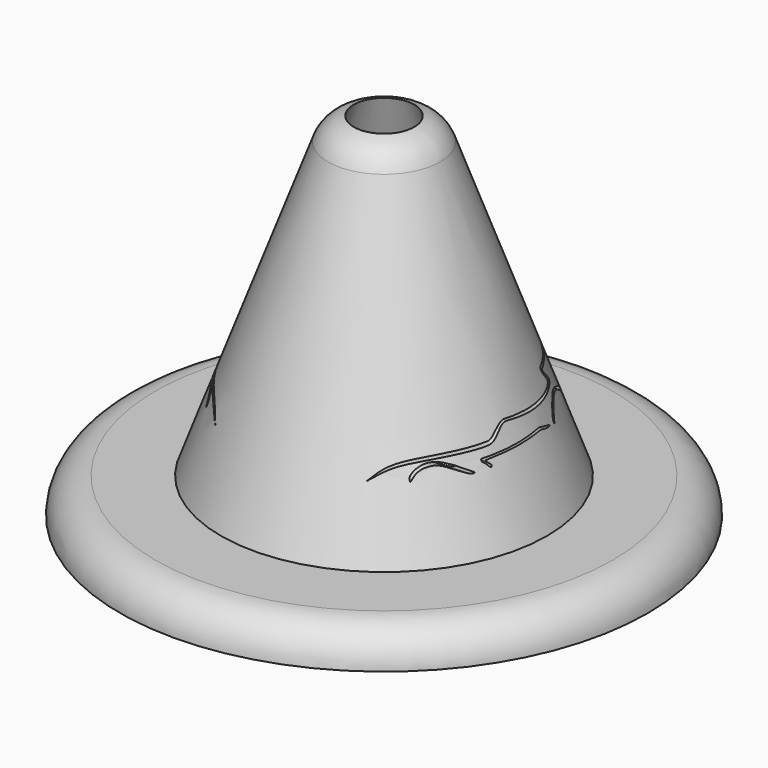
from build123d import *

# Parameters (mm, degrees)
F0_R          = 50
F0_R_2        = 45
F1_DEPTH      = 100
F1_TAPER      = 20
F2_DEPTH      = 100
F2_TAPER      = 20
F0_R_3        = 75
F3_DEPTH      = 10
F3_TAPER      = -20
F5_DEPTH      = 40
F5_DEPTH_BACK = 40


# Not quite as in the source:
# - a fillet or chamfer that OpenCascade refuses, or shapes differently, is made with other operations: its cross-section is extruded or revolved along the edge and cut away or added


with BuildPart() as f1:
    # F0 (on Top) → F1 (new body)
    with BuildSketch(Plane.XY):
        Circle(F0_R)
        Circle(F0_R_2, mode=Mode.SUBTRACT)
        Circle(F0_R_2)
    extrude(amount=F1_DEPTH, taper=F1_TAPER)

    # F0 (on Top) → F2 (cut)
    with BuildSketch(Plane.XY):
        Circle(F0_R_2)
    extrude(amount=F2_DEPTH, taper=F2_TAPER, mode=Mode.SUBTRACT)

    # F0 (on Top) → F3 (join)
    with BuildSketch(Plane.XY):
        Circle(F0_R_3)
        Circle(F0_R, mode=Mode.SUBTRACT)
    extrude(amount=F3_DEPTH, taper=F3_TAPER)

    # F4 (on Right) → F5 (cut, two sides)
    with BuildSketch(Plane.YZ) as f5_sk:
        with BuildLine():
            add(Edge.make_bspline(
                [(-33.0905122474, 29.0107644992), (-32.4736289516, 29.4855445157), (-31.0186418233, 30.6053652357), (-26.9459934351, 33.0948601121), (-14.7801623352, 33.2154481172), (-8.672900368, 33.0818885283), (-7.3010598226, 33.623406531), (-5.7671409301, 34.7695034497), (-3.603350549, 36.7572104234), (-1.1111195238, 36.4115912996), (5.5015940536, 35.4228440969), (10.74246847, 35.0882430818), (15.6437072481, 34.987577792), (20.8910014478, 35.7164902028), (18.1980442225, 37.9974433258), (16.9738401589, 39.7907033697), (17.7865173787, 39.7330347723), (20.0394734839, 39.7776412616), (26.3179551973, 39.6554872999), (30.4444185386, 40.2482755124), (32.5263710484, 40.5470123977)],
                knots=[0, 0, 0, 0, 0.0451475883, 0.1069196297, 0.2094003196, 0.2800605832, 0.3124517037, 0.3521408548, 0.3999822498, 0.4445315809, 0.5189515251, 0.5865582039, 0.6536105299, 0.7088728063, 0.7541204751, 0.7934668639, 0.8112489161, 0.8536560226, 0.926473828, 1, 1, 1, 1], degree=3))
            add(Edge.make_bspline(
                [(32.5263710484, 40.5470123977), (30.1976356747, 40.4635342007), (25.2690463426, 40.2868590164), (19.4529417348, 40.396089847), (16.3849193114, 40.4537096218)],
                knots=[0, 0, 0, 0, 0.472495316, 1, 1, 1, 1], degree=3))
            add(Edge.make_bspline(
                [(16.3849193114, 40.4537096218), (16.5686048113, 39.7383730029), (16.9565205292, 38.3150686964), (21.4343349953, 34.8701721906), (7.4818398942, 35.9873174196), (-3.2351667173, 37.2132535267)],
                knots=[0, 0, 0, 0, 0.1993748097, 0.391377201, 1, 1, 1, 1], degree=3))
            add(Edge.make_bspline(
                [(-3.2351667173, 37.2132535267), (-5.9701177432, 36.3668073114), (-6.9092386051, 34.5355377436), (-8.6203338758, 34.1090930525)],
                knots=[0, 0, 0, 0, 6.2157732885, 6.2157732885, 6.2157732885, 6.2157732885], degree=3))
            add(Edge.make_bspline(
                [(-8.6203338758, 34.1090930525), (-14.5863803397, 33.8637664695), (-27.6658774108, 34.5977789594), (-31.4557963438, 30.6431434265), (-33.0905122474, 29.0107644992)],
                knots=[0, 0, 0, 0, 0.618362291, 1, 1, 1, 1], degree=3))
        make_face()
        with BuildLine():
            add(Edge.make_bspline(
                [(-26.909318541, 28.6785699918), (-26.8956395308, 29.0550856543), (-26.8601785209, 30.0311523057), (-24.3210936276, 32.293186642), (-20.5030238961, 32.9063750111), (-16.421347657, 30.179098201), (-13.9781577953, 28.5466181457)],
                knots=[0, 0, 0, 0, 0.1464289315, 0.3795974805, 0.6286424848, 1, 1, 1, 1], degree=3))
            add(Edge.make_bspline(
                [(-13.9781577953, 28.5466181457), (-14.2737865515, 28.4716503343), (-15.2163200417, 28.2326354499), (-19.7471855154, 31.2612430572), (-22.0542026714, 31.9048500684), (-25.0846623627, 31.1021368623), (-26.2937481092, 29.4961903866), (-26.909318541, 28.6785699918)],
                knots=[0, 0, 0, 0, 0.1254845549, 0.4000740558, 0.5918971887, 0.7922264616, 1, 1, 1, 1], degree=3))
        make_face()
        with BuildLine():
            add(Edge.make_bspline(
                [(-9.9345830013, 28.6598701102), (-10.2675818403, 28.7198319859), (-10.9003286687, 29.9244436138), (-11.7667029195, 30.1550577471), (-11.7303005199, 30.9825030934), (-11.1805494134, 30.9455152519), (7.8860175685, 31.2394349499), (7.5029550194, 31.2710197722), (13.3797988078, 29.5980368417), (11.1528119969, 29.6089395606), (8.1590386099, 30.5150460799), (7.7765984584, 30.6470446813), (-10.7555014846, 30.5645954508), (-10.7132201965, 30.3452443993), (-10.7949253185, 30.0675032085), (-9.2597765347, 29.0612951912), (-9.7549917724, 28.6275317784), (-9.9345830013, 28.6598701102)],
                knots=[0, 0, 0, 0, 0.0574162707, 0.1006189695, 0.1351088035, 0.168735216, 0.3685417337, 0.4055091331, 0.5050900385, 0.5473015241, 0.628784027, 0.6826490599, 0.8788117099, 0.8897597101, 0.9105480692, 0.9690345509, 1, 1, 1, 1], degree=3))
        make_face()
        with BuildLine():
            add(Edge.make_bspline(
                [(14.7013281602, 28.6206390895), (14.6405472638, 29.0722058099), (14.4989867185, 30.1239183553), (16.2352054341, 32.0087749061), (18.8620217309, 33.7182216009), (21.9139736425, 33.7315879037), (26.9762607989, 30.6280239128), (30.3145315813, 28.5814120411)],
                knots=[0, 0, 0, 0, 0.126477424, 0.2945697447, 0.4823409145, 0.6586352874, 1, 1, 1, 1], degree=3))
            add(Edge.make_bspline(
                [(14.7013281602, 28.6206390895), (14.8536817826, 28.9647850713), (15.2086946587, 29.766710571), (16.6304101619, 31.3410571251), (19.0593933628, 33.1075353098), (22.0411489581, 33.015227137), (26.9394300692, 29.7010386456), (27.8872859724, 28.9135223535), (29.4282801304, 28.7026742838), (30.3145315813, 28.5814120411)],
                knots=[0, 0, 0, 0, 0.0992735502, 0.2313262266, 0.3844956235, 0.5405621256, 0.7575190051, 0.8605451342, 1, 1, 1, 1], degree=3))
        make_face()
    extrude(amount=F5_DEPTH, mode=Mode.SUBTRACT)
    extrude(f5_sk.sketch, amount=-F5_DEPTH_BACK, mode=Mode.SUBTRACT)

    # F6: fillet of radius 10 on 2 edges, made by hand

    # F6_s1 → F6_t2 (revolve, cut)
    with BuildSketch(Plane.XZ):
        with BuildLine():
            ThreePointArc((8.6029765734, 100), (13.0827890608, 97.765288027), (15.918081832, 93.6393005783))
            Line((15.918081832, 93.6393005783), (13.6029765734, 100))
            Line((13.6029765734, 100), (8.6029765734, 100))
        make_face()
    revolve(axis=Axis((0, 0, 100), (0, 0, -1)), mode=Mode.SUBTRACT)

    # F6_s3 → F6_t4 (revolve, cut)
    with BuildSketch(Plane.XZ):
        with BuildLine():
            ThreePointArc((75, 0), (72.0710678119, 7.0710678119), (65, 10))
            Line((65, 10), (78.6397023427, 10))
            Line((78.6397023427, 10), (75, 0))
        make_face()
    revolve(axis=Axis((0, 0, 10), (0, 0, -1)), mode=Mode.SUBTRACT)


solid = f1.part
